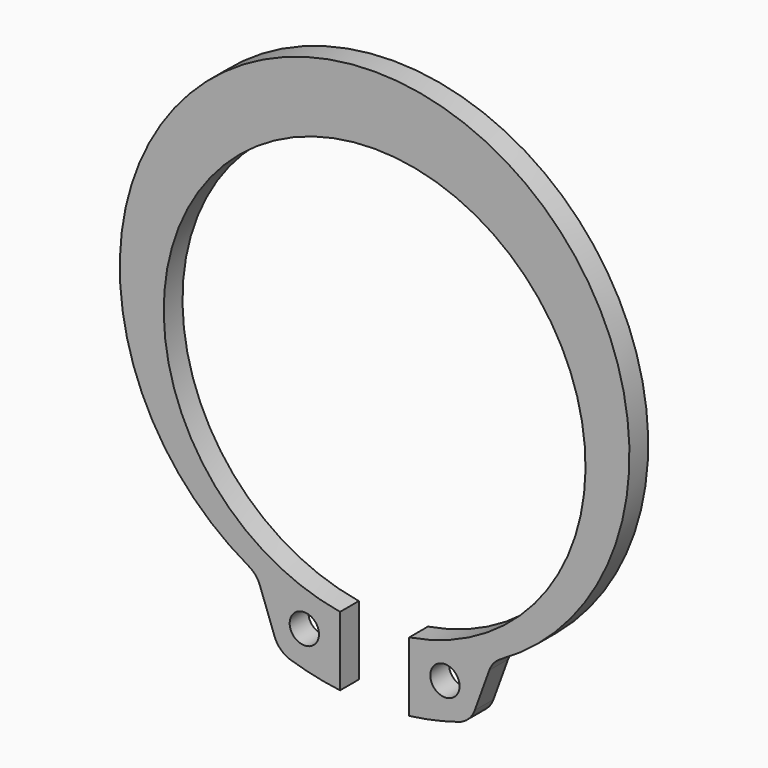
from build123d import *

# Parameters (mm, degrees)
F1_DEPTH = 2
F2_R     = 2.15


# Not quite as in the source:
# - a feature names something its author has since deleted; it is built from what else it names


with BuildPart() as f1:
    # F0 (on Front) → F1 (new body)
    with BuildSketch(Plane.XZ):
        with BuildLine():
            ThreePointArc((-2.95, -17.7566184844), (0, 18), (2.95, -17.7566184844))
            Line((2.95, -17.7566184844), (2.95, -19.4990138986))
            ThreePointArc((2.95, -19.4990138986), (4.0741879212, -19.3150062668), (5.1871999415, -19.0723923069))
            ThreePointArc((5.1871999415, -19.0723923069), (5.6730323101, -18.8149936793), (6.2223129211, -18.7909529991))
            ThreePointArc((6.2223129211, -18.7909529991), (8.1825487808, -18.102131288), (10.0681136131, -17.2294084005))
            ThreePointArc((10.0681136131, -17.2294084005), (0, 23.8), (-10.0681136131, -17.2294084005))
            ThreePointArc((-10.0681136131, -17.2294084005), (-8.1825487808, -18.102131288), (-6.2223129211, -18.7909529991))
            ThreePointArc((-6.2223129211, -18.7909529991), (-5.6730323101, -18.8149936793), (-5.1871999415, -19.0723923069))
            ThreePointArc((-5.1871999415, -19.0723923069), (-4.0741879212, -19.3150062668), (-2.95, -19.4990138986))
            Line((-2.95, -19.4990138986), (-2.95, -17.7566184844))
        make_face()
        with BuildLine():
            ThreePointArc((5.1871999415, -19.0723923069), (4.0741879212, -19.3150062668), (2.95, -19.4990138986))
            Line((2.95, -19.4990138986), (2.95, -23.6566184844))
            ThreePointArc((2.95, -23.6566184844), (5.6060820605, -23.1713172273), (8.1902527715, -22.3887886599))
            Line((8.1902527715, -22.3887886599), (10.0681136131, -17.2294084005))
            ThreePointArc((10.0681136131, -17.2294084005), (8.1825487808, -18.102131288), (6.2223129211, -18.7909529991))
            ThreePointArc((6.2223129211, -18.7909529991), (6.9599367667, -19.2193782076), (7.2509916054, -20.0212037359))
            ThreePointArc((7.2509916054, -20.0212037359), (5.4788515763, -21.1569280818), (5.1871999415, -19.0723923069))
        make_face()
        with BuildLine():
            Line((-2.95, -23.6566184844), (-2.95, -19.4990138986))
            ThreePointArc((-2.95, -19.4990138986), (-4.0741879212, -19.3150062668), (-5.1871999415, -19.0723923069))
            ThreePointArc((-5.1871999415, -19.0723923069), (-4.8652672595, -19.4990637067), (-4.7509916054, -20.0212037359))
            ThreePointArc((-4.7509916054, -20.0212037359), (-6.8028171337, -20.9801488971), (-6.2223129211, -18.7909529991))
            ThreePointArc((-6.2223129211, -18.7909529991), (-8.1825487808, -18.102131288), (-10.0681136131, -17.2294084005))
            Line((-10.0681136131, -17.2294084005), (-8.1902527715, -22.3887886599))
            ThreePointArc((-8.1902527715, -22.3887886599), (-5.6060820605, -23.1713172273), (-2.95, -23.6566184844))
        make_face()
    extrude(amount=F1_DEPTH)

    # F2
    f2_edges = [f1.edges().sort_by_distance(p)[0] for p in [
        (-10.068114, -1, -17.229408),
        (-8.190253, -1, -22.388789),
        (8.190253, -1, -22.388789),
        (10.068114, -1, -17.229408),
    ]]
    fillet(f2_edges, radius=F2_R)


solid = f1.part
